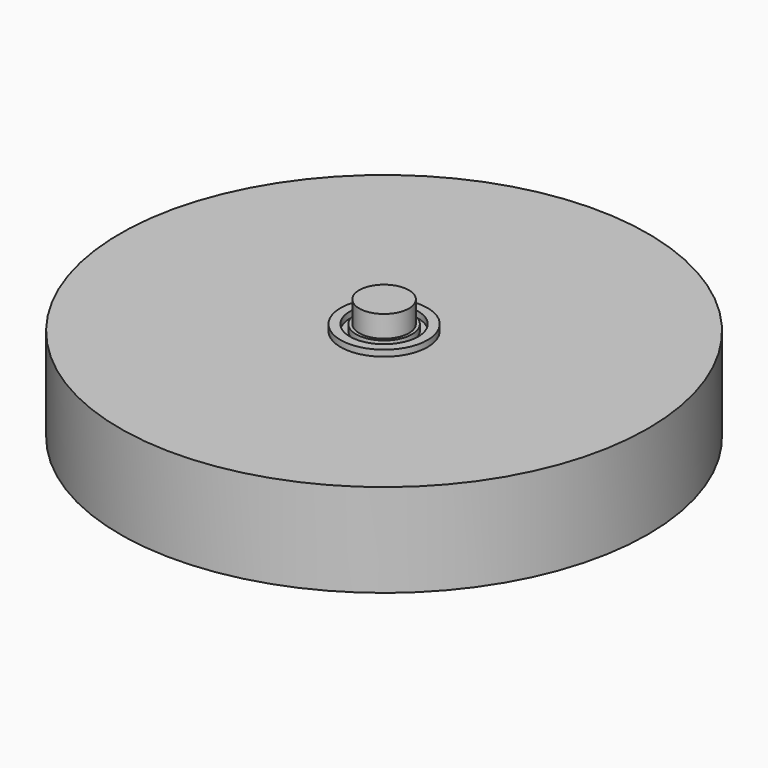
from build123d import *

# Parameters (mm, degrees)
F0_R     = 11
F1_DEPTH = 25
F0_R_2   = 14
F2_DEPTH = 32
F0_R_3   = 50
F3_DEPTH = 25
F4_R     = 8
F5_DEPTH = 39
F4_R_2   = 9
F6_DEPTH = 32
F4_R_3   = 85
F7_DEPTH = 30


with BuildPart() as f1:
    # F0 (on Top) → F1 (new body)
    with BuildSketch(Plane.XY):
        Circle(F0_R)
    extrude(amount=F1_DEPTH)

    # F0 (on Top) → F2 (join)
    with BuildSketch(Plane.XY):
        Circle(F0_R_2)
        Circle(F0_R, mode=Mode.SUBTRACT)
    extrude(amount=F2_DEPTH)

    # F0 (on Top) → F3 (join)
    with BuildSketch(Plane.XY):
        Circle(F0_R_3)
        Circle(F0_R_2, mode=Mode.SUBTRACT)
    extrude(amount=F3_DEPTH)


with BuildPart() as f5:
    # F4 (on Top) → F5 (new body)
    with BuildSketch(Plane.XY):
        Circle(F4_R)
    extrude(amount=F5_DEPTH)

    # F4 (on Top) → F6 (join)
    with BuildSketch(Plane.XY):
        Circle(F4_R_2)
        Circle(F4_R, mode=Mode.SUBTRACT)
    extrude(amount=F6_DEPTH)

    # F4 (on Top) → F7 (join)
    with BuildSketch(Plane.XY):
        Circle(F4_R_3)
        Circle(F4_R_2, mode=Mode.SUBTRACT)
    extrude(amount=F7_DEPTH)


solid = Compound([f1.part, f5.part])
